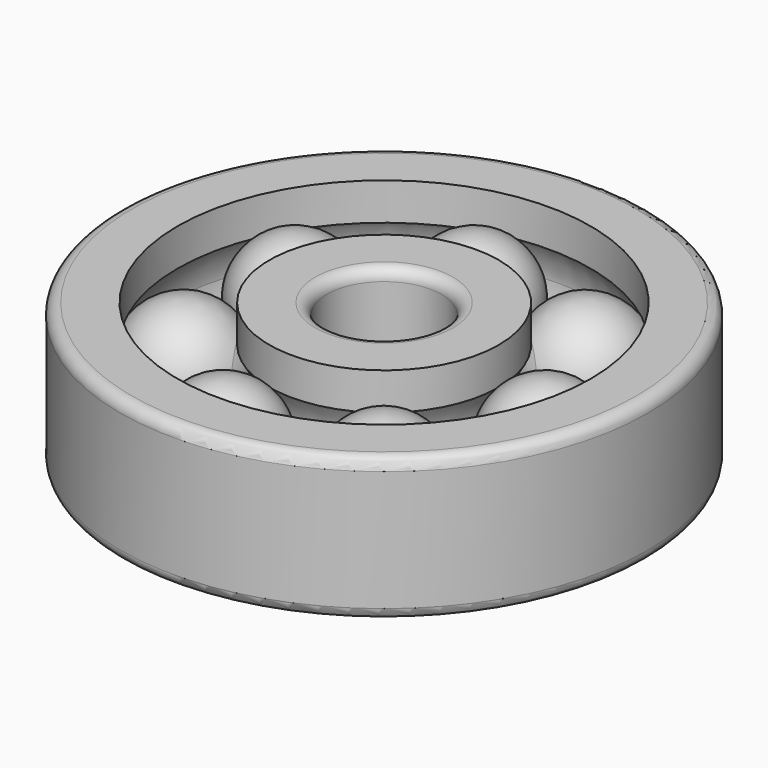
from build123d import *

# Parameters (mm, degrees)
F4_COUNT = 7
F5_R     = 2.54
F5_2_R   = 2.54


# Not quite as in the source:
# - after a boolean that leaves OpenCascade's solid faulty, fix() repairs it


with BuildPart() as f1:
    # F0 (on Front) → F1 (revolve)
    with BuildSketch(Plane.XZ):
        with BuildLine():
            ThreePointArc((22.86, 0), (23.5117221148, 4.0160926284), (25.4, 7.62))
            Line((25.4, 7.62), (25.4, 15.875))
            Line((25.4, 15.875), (12.7, 15.875))
            Line((12.7, 15.875), (12.7, -15.875))
            Line((12.7, -15.875), (25.4, -15.875))
            Line((25.4, -15.875), (25.4, -7.62))
            ThreePointArc((25.4, -7.62), (23.5117221148, -4.0160926284), (22.86, 0))
        make_face()
    revolve(axis=Axis((0, 0, 0), (0, 0, 1)))

    # F5#2
    f5_2_edges = [f1.edges().sort_by_distance(p)[0] for p in [
        (-12.7, 0, 15.875),
        (-12.7, 0, -15.875),
    ]]
    fillet(f5_2_edges, radius=F5_2_R)


with BuildPart() as f2:
    # F0 (on Front) → F2 (revolve)
    with BuildSketch(Plane.XZ):
        with BuildLine():
            ThreePointArc((45.72, 7.62), (47.6082778852, 4.0160926284), (48.26, 0))
            ThreePointArc((48.26, 0), (47.6082778852, -4.0160926284), (45.72, -7.62))
            Line((45.72, -7.62), (45.72, -15.875))
            Line((45.72, -15.875), (58.42, -15.875))
            Line((58.42, -15.875), (58.42, 15.875))
            Line((58.42, 15.875), (45.72, 15.875))
            Line((45.72, 15.875), (45.72, 7.62))
        make_face()
    revolve(axis=Axis((0, 0, 0), (0, 0, 1)))

    # F5
    f5_edges = [f2.edges().sort_by_distance(p)[0] for p in [
        (-58.42, 0, 15.875),
        (-58.42, 0, -15.875),
    ]]
    fillet(f5_edges, radius=F5_R)


with BuildPart() as f3:
    # F0 (on Front) → F3 (revolve)
    with BuildSketch(Plane.XZ):
        with BuildLine():
            ThreePointArc((45.72, -7.62), (47.6082778852, -4.0160926284), (48.26, 0))
            Line((48.26, 0), (45.72, 0))
            Line((45.72, 0), (45.72, -7.62))
        make_face()
        with BuildLine():
            Line((45.72, 0), (45.72, 7.62))
            ThreePointArc((45.72, 7.62), (35.56, 12.7), (25.4, 7.62))
            Line((25.4, 7.62), (25.4, 0))
            Line((25.4, 0), (45.72, 0))
        make_face()
        with BuildLine():
            ThreePointArc((22.86, 0), (23.5117221148, -4.0160926284), (25.4, -7.62))
            Line((25.4, -7.62), (25.4, 0))
            Line((25.4, 0), (22.86, 0))
        make_face()
    revolve(axis=Axis((35.56, 0, 0), (1, 0, 0)))

    add(f3.part.fix(), mode=Mode.REPLACE)


with BuildPart() as f4_1:
    # F4: instance of F3
    add(f3.part.rotate(Axis((0, 0, 0), (0, 0, 1)), 1 * 360 / F4_COUNT))


with BuildPart() as f4_2:
    # F4: instance of F3
    add(f3.part.rotate(Axis((0, 0, 0), (0, 0, 1)), 2 * 360 / F4_COUNT))


with BuildPart() as f4_3:
    # F4: instance of F3
    add(f3.part.rotate(Axis((0, 0, 0), (0, 0, 1)), 3 * 360 / F4_COUNT))


with BuildPart() as f4_4:
    # F4: instance of F3
    add(f3.part.rotate(Axis((0, 0, 0), (0, 0, 1)), 4 * 360 / F4_COUNT))


with BuildPart() as f4_5:
    # F4: instance of F3
    add(f3.part.rotate(Axis((0, 0, 0), (0, 0, 1)), 5 * 360 / F4_COUNT))


with BuildPart() as f4_6:
    # F4: instance of F3
    add(f3.part.rotate(Axis((0, 0, 0), (0, 0, 1)), 6 * 360 / F4_COUNT))


solid = Compound([f1.part, f2.part, f3.part, f4_1.part, f4_2.part, f4_3.part, f4_4.part, f4_5.part, f4_6.part])
